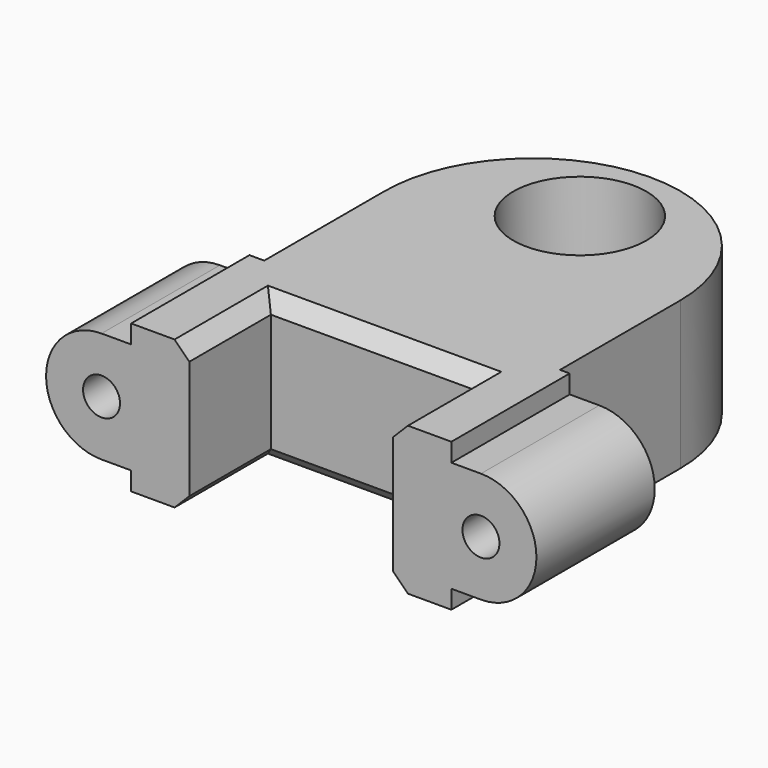
from build123d import *

# Parameters (mm, degrees)
F1_DEPTH = 25.4
F2_R     = 3.175
F3_DEPTH = 25.4
F5_R     = 11.43
F6_DEPTH = 17.78
F7_SIZE  = 2.54


with BuildPart() as f1:
    # F0 (on Top) → F1 (new body)
    with BuildSketch(Plane.XY):
        with BuildLine():
            Line((-24.96, 25.4), (25.8360511508, 25.4))
            Line((25.8360511508, 25.4), (25.8360511508, 51.2478682217))
            ThreePointArc((25.8360511508, 51.2478682217), (0.2121083359, 76.6468809902), (-24.96, 50.8))
            Line((-24.96, 50.8), (-24.96, 25.4))
        make_face()
        Polygon((-17.5, 17.5), (17.5, 17.5), (17.5, 0), (27.5, 0), (27.5, 25.4), (25.8360511508, 25.4), (-24.96, 25.4), (-27.5, 25.4), (-27.5, 0), (-17.5, 0), align=None)
    extrude(amount=F1_DEPTH)



with BuildPart() as f3:
    # F2 (on Front) → F3 (new body)
    with BuildSketch(Plane.XZ):
        with BuildLine():
            Line((-27.5, 3.175), (-27.5, 22.225))
            Line((-27.5, 22.225), (-32.58, 22.225))
            ThreePointArc((-32.58, 22.225), (-42.105, 12.7), (-32.58, 3.175))
            Line((-32.58, 3.175), (-27.5, 3.175))
        make_face()
        with Locations((-32.58, 12.7)):
            Circle(F2_R, mode=Mode.SUBTRACT)
    extrude(amount=-F3_DEPTH)


with BuildPart() as f1_1:
    add(f1.part)

    add(f3.part)  # F4 merges F3
    # F4: F3 across plane
    add(f3.part.mirror(Plane.YZ))

    # F5 (on face) → F6 (cut)
    with BuildSketch(Plane.XY.offset(25.4)):
        with Locations((0, 61.95)):
            Circle(F5_R)
    extrude(amount=-F6_DEPTH, mode=Mode.SUBTRACT)

    # F7
    f7_edges = [f1_1.edges().sort_by_distance(p)[0] for p in [
        (0, 17.5, 25.4),
        (17.5, 8.75, 25.4),
        (-17.5, 8.75, 25.4),
        (17.5, 8.75, 0),
        (0, 17.5, 0),
        (-17.5, 8.75, 0),
    ]]
    chamfer(f7_edges, length=F7_SIZE)


solid = f1_1.part
